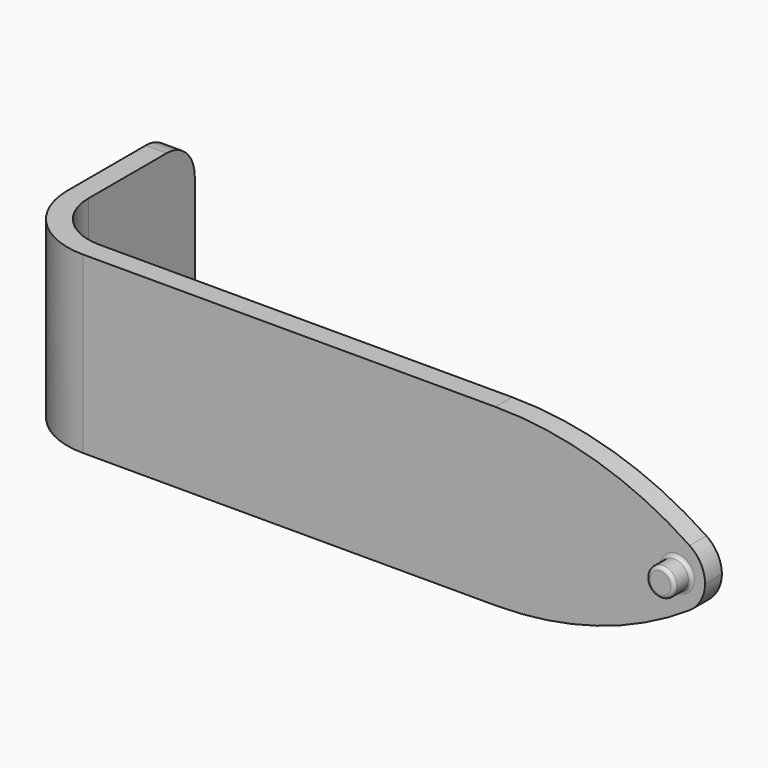
from build123d import *

# Parameters (mm, degrees)
F1_DEPTH     = 25
F2_R         = 2
F3_DEPTH     = 3
F4_SIZE      = 10
F5_T1_DEPTH  = 103
F6_T1_DEPTH  = 16.6158512413
F7_R         = 0.5
F8_R         = 5
F9_TEXT_SIZE = 11.1111111111
F10_DEPTH    = 1


# Not quite as in the source:
# - a fillet or chamfer that OpenCascade refuses, or shapes differently, is made with other operations: its cross-section is extruded or revolved along the edge and cut away or added
# - Text() gives the source's letters only with a copy of the font that has no kerning and outlines rounded to 1/6400 em; it was checked with that copy


with BuildPart() as f1:
    # F0 (on Top) → F1 (new body)
    with BuildSketch(Plane.XY):
        with BuildLine():
            ThreePointArc((0, 11), (3.2218254069, 3.2218254069), (11, 0))
            Line((11, 0), (100, 0))
            Line((100, 0), (100, 3))
            Line((100, 3), (11, 3))
            ThreePointArc((11, 3), (5.3431457505, 5.3431457505), (3, 11))
            Line((3, 11), (3, 30))
            Line((3, 30), (0, 30))
            Line((0, 30), (0, 11))
        make_face()
    extrude(amount=F1_DEPTH)

    # F2 (on face) → F3 (join)
    with BuildSketch(Plane.XZ):
        with Locations((96, 12.5)):
            Circle(F2_R)
    extrude(amount=F3_DEPTH)

    # F4
    f4_edges = [f1.edges().sort_by_distance(p)[0] for p in [
        (100, 1.5, 25),
        (100, 1.5, 0),
    ]]
    chamfer(f4_edges, length=F4_SIZE)

    # F5: fillet of radius 50 on 2 edges, made by hand

    # F5_s2 → F5_t1 (cut)
    with BuildSketch(Plane.XZ.offset(-53)):
        with BuildLine():
            ThreePointArc((70, 25), (85.8113883008, 22.4341649025), (100, 15))
            Line((100, 15), (90, 25))
            Line((90, 25), (70, 25))
        make_face()
        with BuildLine():
            ThreePointArc((70, 0), (85.8113883008, 2.5658350975), (100, 10))
            Line((100, 10), (90, 0))
            Line((90, 0), (70, 0))
        make_face()
    extrude(amount=F5_T1_DEPTH, mode=Mode.SUBTRACT)

    # F6: fillet of radius 5 on 2 edges, made by hand

    # F6_s2 → F6_t1 (cut)
    with BuildSketch(Plane.XZ.offset(-9.8079256207)):
        with BuildLine():
            ThreePointArc((100, 12.4165738677), (99.4095855184, 14.7735964717), (97.7777777778, 16.5739709642))
            ThreePointArc((97.7777777778, 16.5739709642), (98.8996063534, 15.8021170115), (100, 15))
            Line((100, 15), (100, 12.4165738677))
        make_face()
        with BuildLine():
            ThreePointArc((97.7777777778, 8.4260290358), (99.4095855184, 10.2264035283), (100, 12.5834261323))
            Line((100, 12.5834261323), (100, 10))
            ThreePointArc((100, 10), (98.8996063534, 9.1978829885), (97.7777777778, 8.4260290358))
        make_face()
    extrude(amount=F6_T1_DEPTH, mode=Mode.SUBTRACT)

    # F7
    f7_edges = [f1.edges().sort_by_distance(p)[0] for p in [
        (94, 0, 12.5),
        (94, -3, 12.5),
    ]]
    fillet(f7_edges, radius=F7_R)

    # F8
    f8_edges = [f1.edges().sort_by_distance(p)[0] for p in [
        (1.5, 30, 25),
        (1.5, 30, 0),
    ]]
    fillet(f8_edges, radius=F8_R)

    # F9 (on face) → F10 (cut, symmetric)
    with BuildSketch(Plane(origin=(0, 3, 0), x_dir=(-1, 0, 0), z_dir=(0, 1, 0))):
        with Locations((-64.984375, 8.5)):
            Text('H3DS.DJ', F9_TEXT_SIZE, font='Open Sans', font_style=FontStyle.BOLD, text_align=(TextAlign.LEFT, TextAlign.BOTTOM))
    extrude(amount=F10_DEPTH, both=True, mode=Mode.SUBTRACT)


solid = f1.part
